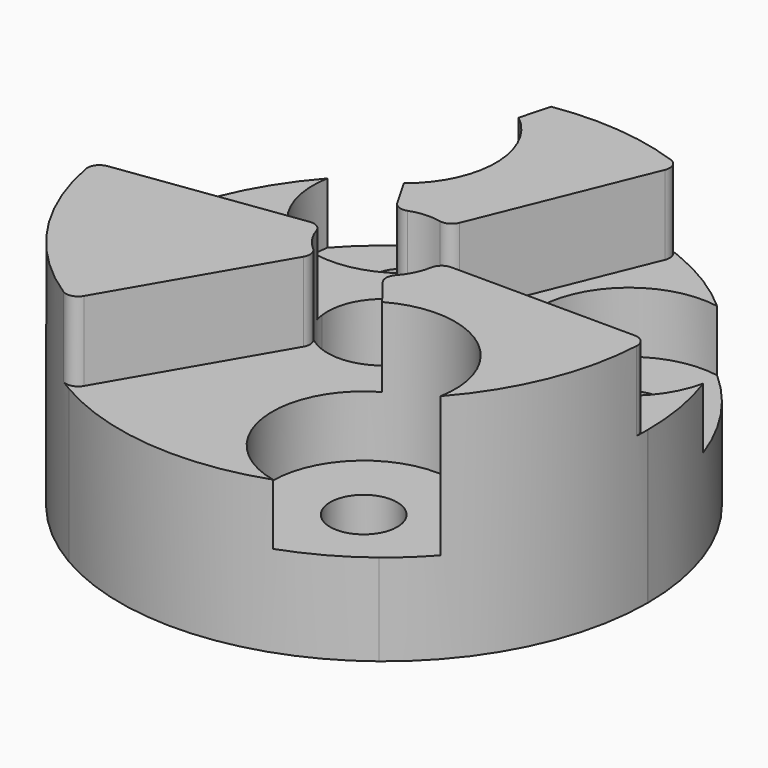
from build123d import *

# Parameters (mm, degrees)
F1_DEPTH      = 3.302
F2_DEPTH      = 6.35
F3_T1_DEPTH   = 4.6338919233
F4_T1_DEPTH   = 4.4582047696
F5_R          = 1.397
F6_DEPTH      = 6.351
F6_DEPTH_BACK = 25.4
F7_R          = 3.81
F8_DEPTH      = 5.842
F9_T1_DEPTH   = 8.456355204
F9_T3_DEPTH   = 2.54


# Not quite as in the source:
# - a fillet or chamfer that OpenCascade refuses, or shapes differently, is made with other operations: its cross-section is extruded or revolved along the edge and cut away or added


with BuildPart() as f1:
    # F0 (on Top) → F1 (new body)
    with BuildSketch(Plane.XY):
        with BuildLine():
            Line((0.8864303251, 2.1758656964), (4.1494522244, 10.1854037464))
            ThreePointArc((4.1494522244, 10.1854037464), (-0.7354841661, 10.9735803766), (-5.4715498037, 9.5405736717))
            Line((-5.4715498037, 9.5405736717), (-1.1688645655, 2.0381133132))
            ThreePointArc((-1.1688645655, 2.0381133132), (-0.157118442, 2.3442406116), (0.8864303251, 2.1758656964))
        make_face()
    extrude(amount=F1_DEPTH)



with BuildPart() as f1b:
    # F0 (on Top) → F1, piece 2 (new body)
    with BuildSketch(Plane.XY):
        with BuildLine():
            Line((-2.3275701308, -0.320261668), (-10.8955445044, -1.4991708351))
            ThreePointArc((-10.8955445044, -1.4991708351), (-9.1356572935, -6.1237381602), (-5.5266042645, -9.5087879639))
            Line((-5.5266042645, -9.5087879639), (-1.1806256223, -2.0313230639))
            ThreePointArc((-1.1806256223, -2.0313230639), (-1.9516127013, -1.3081888679), (-2.3275701308, -0.320261668))
        make_face()
    extrude(amount=F1_DEPTH)


with BuildPart() as f1c:
    # F0 (on Top) → F1, piece 3 (new body)
    with BuildSketch(Plane.XY):
        with BuildLine():
            ThreePointArc((6.74609228, -8.6862329113), (9.8711414597, -4.8498422164), (10.9981540682, -0.0317857078))
            Line((10.9981540682, -0.0317857078), (2.3494901878, -0.0067902494))
            ThreePointArc((2.3494901878, -0.0067902494), (2.1087311432, -1.0360517437), (1.4411398058, -1.8556040284))
            Line((1.4411398058, -1.8556040284), (6.74609228, -8.6862329113))
        make_face()
    extrude(amount=F1_DEPTH)


with BuildPart() as f1_1:
    add(f1.part)

    add(f1b.part)  # F2 merges F1b

    add(f1c.part)  # F2 merges F1c
    # F0 (on Top) → F2 (join)
    with BuildSketch(Plane.XY):
        with BuildLine():
            ThreePointArc((10.9981540682, -0.0317857078), (10.9981885171, -0.0158928705), (10.9982, 0))
            ThreePointArc((10.9982, 0), (9.1267986911, 6.136933183), (4.1494522244, 10.1854037464))
            Line((4.1494522244, 10.1854037464), (0.8864303251, 2.1758656964))
            ThreePointArc((0.8864303251, 2.1758656964), (1.9497202747, 1.3110076661), (2.3495, 0))
            ThreePointArc((2.3495, 0), (2.3494975469, -0.0033951282), (2.3494901878, -0.0067902494))
            Line((2.3494901878, -0.0067902494), (10.9981540682, -0.0317857078))
        make_face()
        with BuildLine():
            Line((0.8864303251, 2.1758656964), (4.1494522244, 10.1854037464))
            ThreePointArc((4.1494522244, 10.1854037464), (-0.7354841661, 10.9735803766), (-5.4715498037, 9.5405736717))
            Line((-5.4715498037, 9.5405736717), (-1.1688645655, 2.0381133132))
            ThreePointArc((-1.1688645655, 2.0381133132), (-0.157118442, 2.3442406116), (0.8864303251, 2.1758656964))
        make_face()
        with BuildLine():
            ThreePointArc((6.74609228, -8.6862329113), (9.8711414597, -4.8498422164), (10.9981540682, -0.0317857078))
            Line((10.9981540682, -0.0317857078), (2.3494901878, -0.0067902494))
            ThreePointArc((2.3494901878, -0.0067902494), (2.1087311432, -1.0360517437), (1.4411398058, -1.8556040284))
            Line((1.4411398058, -1.8556040284), (6.74609228, -8.6862329113))
        make_face()
        with BuildLine():
            Line((-1.1688645655, 2.0381133132), (-5.4715498037, 9.5405736717))
            ThreePointArc((-5.4715498037, 9.5405736717), (-9.8711414597, 4.8498422164), (-10.8955445044, -1.4991708351))
            Line((-10.8955445044, -1.4991708351), (-2.3275701308, -0.320261668))
            ThreePointArc((-2.3275701308, -0.320261668), (-2.1087311432, 1.0360517437), (-1.1688645655, 2.0381133132))
        make_face()
        with BuildLine():
            ThreePointArc((-5.5266042645, -9.5087879639), (0.7354841661, -10.9735803766), (6.74609228, -8.6862329113))
            Line((6.74609228, -8.6862329113), (1.4411398058, -1.8556040284))
            ThreePointArc((1.4411398058, -1.8556040284), (0.157118442, -2.3442406116), (-1.1806256223, -2.0313230639))
            Line((-1.1806256223, -2.0313230639), (-5.5266042645, -9.5087879639))
        make_face()
        with BuildLine():
            Line((-2.3275701308, -0.320261668), (-10.8955445044, -1.4991708351))
            ThreePointArc((-10.8955445044, -1.4991708351), (-9.1356572935, -6.1237381602), (-5.5266042645, -9.5087879639))
            Line((-5.5266042645, -9.5087879639), (-1.1806256223, -2.0313230639))
            ThreePointArc((-1.1806256223, -2.0313230639), (-1.9516127013, -1.3081888679), (-2.3275701308, -0.320261668))
        make_face()
    extrude(amount=-F2_DEPTH)

    # F3: fillet of radius 0.508 on 6 edges, made by hand

    # F3_s2 → F3_t1 (cut)
    with BuildSketch(Plane.XY):
        with BuildLine():
            ThreePointArc((3.9531481969, 9.7035483908), (3.9459668292, 10.1036299064), (3.6513440541, 10.3743958782))
            ThreePointArc((3.6513440541, 10.3743958782), (3.901542663, 10.2829163222), (4.1494522244, 10.1854037464))
            Line((4.1494522244, 10.1854037464), (3.9531481969, 9.7035483908))
        make_face()
        with BuildLine():
            ThreePointArc((10.9837113978, -0.5643466757), (10.8451967866, -0.1889395718), (10.4778487793, -0.0302819762))
            Line((10.4778487793, -0.0302819762), (10.9981540682, -0.0317857078))
            ThreePointArc((10.9981540682, -0.0317857078), (10.9941578867, -0.2981536556), (10.9837113978, -0.5643466757))
        make_face()
        with BuildLine():
            ThreePointArc((-5.212699429, 9.089224208), (-5.2589719244, 9.4866857122), (-5.0031171412, 9.7943464361))
            ThreePointArc((-5.0031171412, 9.7943464361), (-5.2388703034, 9.6702968509), (-5.4715498037, 9.5405736717))
            Line((-5.4715498037, 9.5405736717), (-5.212699429, 9.089224208))
        make_face()
        with BuildLine():
            ThreePointArc((7.1588183524, -8.3493546479), (6.7770167548, -8.4691224698), (6.4269453148, -8.2753009589))
            Line((6.4269453148, -8.2753009589), (6.74609228, -8.6862329113))
            ThreePointArc((6.74609228, -8.6862329113), (6.9544954285, -8.5202932212), (7.1588183524, -8.3493546479))
        make_face()
        with BuildLine():
            ThreePointArc((-5.9805942565, -9.2299997605), (-5.5862248623, -9.2977461404), (-5.2651493503, -9.0589422318))
            Line((-5.2651493503, -9.0589422318), (-5.5266042645, -9.5087879639))
            ThreePointArc((-5.5266042645, -9.5087879639), (-5.7552875833, -9.3721431953), (-5.9805942565, -9.2299997605))
        make_face()
        with BuildLine():
            ThreePointArc((-10.3800935118, -1.428247432), (-10.722983584, -1.6345074366), (-10.8101624065, -2.0250412303))
            ThreePointArc((-10.8101624065, -2.0250412303), (-10.8560380915, -1.762623101), (-10.8955445044, -1.4991708351))
            Line((-10.8955445044, -1.4991708351), (-10.3800935118, -1.428247432))
        make_face()
    extrude(amount=F3_T1_DEPTH, mode=Mode.SUBTRACT)

    # F4: fillet of radius 0.508 on 6 edges, made by hand

    # F4_s2 → F4_t1 (cut)
    with BuildSketch(Plane.XY):
        with BuildLine():
            ThreePointArc((-2.7857353042, -0.3833028373), (-2.4469491553, -0.4559663275), (-2.2335580647, -0.7289503561))
            ThreePointArc((-2.2335580647, -0.7289503561), (-2.2897006824, -0.5267077321), (-2.3275701308, -0.320261668))
            Line((-2.3275701308, -0.320261668), (-2.7857353042, -0.3833028373))
        make_face()
        with BuildLine():
            ThreePointArc((-1.5229431343, -1.7890764264), (-1.3515120564, -2.0901867434), (-1.4130231496, -2.4311741667))
            Line((-1.4130231496, -2.4311741667), (-1.1806256223, -2.0313230639))
            ThreePointArc((-1.1806256223, -2.0313230639), (-1.3572000088, -1.9178525455), (-1.5229431343, -1.7890764264))
        make_face()
        with BuildLine():
            ThreePointArc((-0.7879140674, 2.2134456561), (-1.1343987902, 2.215537146), (-1.3989470146, 2.439301027))
            Line((-1.3989470146, 2.439301027), (-1.1688645655, 2.0381133132))
            ThreePointArc((-1.1688645655, 2.0381133132), (-0.9823090207, 2.1342959584), (-0.7879140674, 2.2134456561))
        make_face()
        with BuildLine():
            ThreePointArc((0.4854895058, 2.2987932029), (0.8285961548, 2.3471032941), (1.0609176577, 2.6041689603))
            Line((1.0609176577, 2.6041689603), (0.8864303251, 2.1758656964))
            ThreePointArc((0.8864303251, 2.1758656964), (0.6887080648, 2.2462928241), (0.4854895058, 2.2987932029))
        make_face()
        with BuildLine():
            ThreePointArc((1.7248176465, -2.220866123), (1.6183530006, -1.8911369665), (1.7480685589, -1.5698428468))
            ThreePointArc((1.7480685589, -1.5698428468), (1.6009926176, -1.719585092), (1.4411398058, -1.8556040284))
            Line((1.4411398058, -1.8556040284), (1.7248176465, -2.220866123))
        make_face()
        with BuildLine():
            ThreePointArc((2.8119701642, -0.0081268603), (2.4859108466, -0.1253504027), (2.3108572018, -0.4243692296))
            ThreePointArc((2.3108572018, -0.4243692296), (2.3395090295, -0.2164434129), (2.3494901878, -0.0067902494))
            Line((2.3494901878, -0.0067902494), (2.8119701642, -0.0081268603))
        make_face()
    extrude(amount=F4_T1_DEPTH, mode=Mode.SUBTRACT)

    # F5 (on face) → F6 (cut, two sides)
    with BuildSketch(Plane.XY) as f6_sk:
        with Locations((-4.4645385024, 6.6395705404)):
            Circle(F5_R)
        with Locations((6.6395705404, 4.4645385024)):
            Circle(F5_R)
        with Locations((4.4645385024, -6.6395705404)):
            Circle(F5_R)
    extrude(amount=-F6_DEPTH, mode=Mode.SUBTRACT)
    extrude(f6_sk.sketch, amount=F6_DEPTH_BACK, mode=Mode.SUBTRACT)

    # F7 (on face) → F8 (cut)
    with BuildSketch(Plane.XY.offset(3.302)):
        with Locations((4.4645385024, -6.6395705404)):
            Circle(F7_R)
        with Locations((6.6395705404, 4.4645385024)):
            Circle(F7_R)
        with BuildLine():
            ThreePointArc((-2.0962074568, 3.6550926868), (-1.0338358569, 4.9823501693), (-0.6545385024, 6.6395705404))
            ThreePointArc((-0.6545385024, 6.6395705404), (-1.5039813545, 9.0377367927), (-3.6735418484, 10.3665564933))
            ThreePointArc((-3.6735418484, 10.3665564933), (-4.3477533155, 10.102348457), (-5.0031171412, 9.7943464361))
            ThreePointArc((-5.0031171412, 9.7943464361), (-5.2589719244, 9.4866857122), (-5.212699429, 9.089224208))
            Line((-5.212699429, 9.089224208), (-4.6049424864, 8.0294970569))
            ThreePointArc((-4.6049424864, 8.0294970569), (-3.5276648091, 7.6758507548), (-3.0675385024, 6.6395705404))
            ThreePointArc((-3.0675385024, 6.6395705404), (-3.1362873981, 6.2067218326), (-3.3357675701, 5.8164756598))
            Line((-3.3357675701, 5.8164756598), (-2.0962074568, 3.6550926868))
        make_face()
        with BuildLine():
            ThreePointArc((-5.0031171412, 9.7943464361), (-4.3477533155, 10.102348457), (-3.6735418484, 10.3665564933))
            ThreePointArc((-3.6735418484, 10.3665564933), (-8.1734837008, 5.7678908314), (-2.0962074568, 3.6550926868))
            Line((-2.0962074568, 3.6550926868), (-3.3357675701, 5.8164756598))
            ThreePointArc((-3.3357675701, 5.8164756598), (-3.1362873981, 6.2067218326), (-3.0675385024, 6.6395705404))
            ThreePointArc((-3.0675385024, 6.6395705404), (-3.5276648091, 7.6758507548), (-4.6049424864, 8.0294970569))
            Line((-4.6049424864, 8.0294970569), (-5.212699429, 9.089224208))
            ThreePointArc((-5.212699429, 9.089224208), (-5.2589719244, 9.4866857122), (-5.0031171412, 9.7943464361))
        make_face()
    extrude(amount=-F8_DEPTH, mode=Mode.SUBTRACT)

    # F9: chamfer of 2.54 on 2 edges, made by hand

    # F9_s2 → F9_t1 (cut)
    with BuildSketch(Plane.XY):
        with BuildLine():
            Line((-1.6990973778, 10.9601467928), (-2.0905864719, 9.5002911113))
            Line((-2.0905864719, 9.5002911113), (-2.1225900483, 9.460839735))
            ThreePointArc((-2.1225900483, 9.460839735), (-2.8366247449, 10.0280040188), (-3.6840884704, 10.3168633472))
            Line((-3.6840884704, 10.3168633472), (-3.6905097091, 10.4144389713))
            ThreePointArc((-3.6905097091, 10.4144389713), (-2.6991406456, 10.7142447599), (-1.7070669555, 11.0103177588))
            Line((-1.7070669555, 11.0103177588), (-1.6990973778, 10.9601467928))
        make_face()
    extrude(amount=F9_T1_DEPTH, mode=Mode.SUBTRACT)

    # F9_s4 → F9_t3 (cut)
    with BuildSketch(Plane.XY.offset(-2.54)):
        with BuildLine():
            Line((-2.0905864719, 9.5002911113), (-1.6990973778, 10.9601467928))
            Line((-1.6990973778, 10.9601467928), (-1.7070669555, 11.0103177588))
            ThreePointArc((-1.7070669555, 11.0103177588), (-2.6991406456, 10.7142447599), (-3.6905097091, 10.4144389713))
            Line((-3.6905097091, 10.4144389713), (-3.6840884704, 10.3168633472))
            ThreePointArc((-3.6840884704, 10.3168633472), (-2.8366247449, 10.0280040188), (-2.1225900483, 9.460839735))
            Line((-2.1225900483, 9.460839735), (-2.0905864719, 9.5002911113))
        make_face()
    extrude(amount=F9_T3_DEPTH, mode=Mode.SUBTRACT)


solid = f1_1.part
